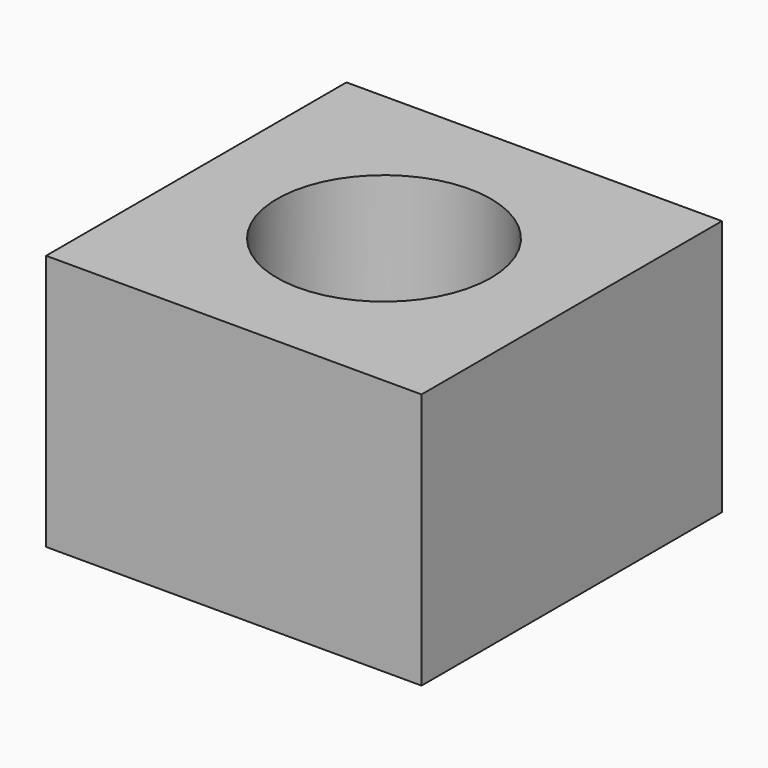
from build123d import *

# Parameters (mm, degrees)
F0_W     = 4.65
F0_H     = 4.65
F0_R     = 1.325
F1_DEPTH = 3.175


# Not quite as in the source:
# - a length typed as a fraction of an inch, garbled in the dataset ("3 / 203.2 mm" for 3/8 in), is restored


with BuildPart() as f1:
    # F0 (on Top) → F1 (new body)
    with BuildSketch(Plane.XY):
        Rectangle(F0_W, F0_H)
        Circle(F0_R, mode=Mode.SUBTRACT)
    extrude(amount=F1_DEPTH)


solid = f1.part
